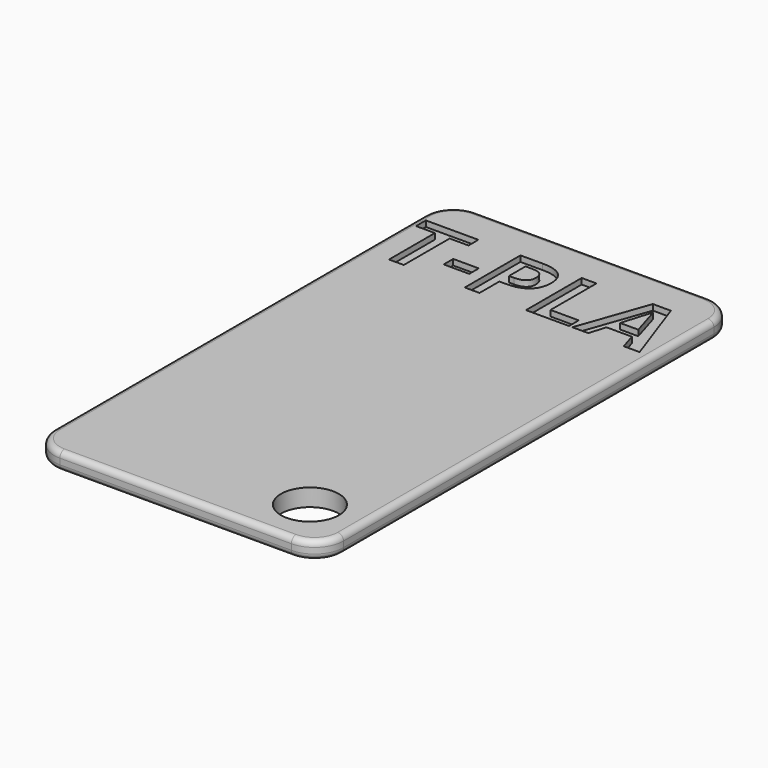
from build123d import *

# Parameters (mm, degrees)
F0_W         = 90
F0_H         = 50
F1_DEPTH     = 3
F2_R         = 1
F3_T1_DEPTH  = 3
F3_T4_ANGLE  = 90
F3_T6_ANGLE  = 90
F3_T8_ANGLE  = 90
F3_T10_ANGLE = 90
F3_T12_ANGLE = 90
F3_T14_ANGLE = 90
F3_T16_ANGLE = 90
F3_T18_ANGLE = 90
F5_ANGLE     = 90
F6_TEXT_SIZE = 16.8504196149
F7_DEPTH     = 1
F8_R         = 5
F9_DEPTH     = 3


# Not quite as in the source:
# - a fillet or chamfer that OpenCascade refuses, or shapes differently, is made with other operations: its cross-section is extruded or revolved along the edge and cut away or added
# - Text() gives the source's letters only with a copy of the font that has no kerning and outlines rounded to 1/6400 em; it was checked with that copy


with BuildPart() as f1:
    # F0 (on Top) → F1 (new body)
    with BuildSketch(Plane.XY):
        Rectangle(F0_W, F0_H)
    extrude(amount=F1_DEPTH)

    # F2
    f2_edges = [f1.edges().sort_by_distance(p)[0] for p in [
        (0, 25, 3),
        (-45, 0, 3),
        (0, -25, 3),
        (45, 0, 3),
        (0, 25, 0),
        (-45, 0, 0),
        (0, -25, 0),
        (45, 0, 0),
    ]]
    fillet(f2_edges, radius=F2_R)

    # F3: fillet of radius 5 on 4 edges, made by hand

    # F3_s2 → F3_t1 (cut)
    with BuildSketch(Plane.XY):
        with BuildLine():
            ThreePointArc((45, -20), (43.5355339059, -23.5355339059), (40, -25))
            Line((40, -25), (45, -25))
            Line((45, -25), (45, -20))
        make_face()
        with BuildLine():
            ThreePointArc((40, 25), (43.5355339059, 23.5355339059), (45, 20))
            Line((45, 20), (45, 25))
            Line((45, 25), (40, 25))
        make_face()
        with BuildLine():
            ThreePointArc((-40, 25), (-43.5355339059, 23.5355339059), (-45, 20))
            Line((-45, 20), (-45, 25))
            Line((-45, 25), (-40, 25))
        make_face()
        with BuildLine():
            ThreePointArc((-45, -20), (-43.5355339059, -23.5355339059), (-40, -25))
            Line((-40, -25), (-45, -25))
            Line((-45, -25), (-45, -20))
        make_face()
    extrude(amount=F3_T1_DEPTH, mode=Mode.SUBTRACT)

    # F3_s3 → F3_t4 (revolve, cut)
    with BuildSketch(Plane.YZ.offset(-40)):
        with BuildLine():
            ThreePointArc((-24, 0), (-24.7071067812, 0.2928932188), (-25, 1))
            Line((-25, 1), (-25, 0))
            Line((-25, 0), (-24, 0))
        make_face()
    revolve(axis=Axis((-40, -20, 0), (0, 0, -1)), revolution_arc=F3_T4_ANGLE, mode=Mode.SUBTRACT)

    # F3_s5 → F3_t6 (revolve, cut)
    with BuildSketch(Plane.XZ.offset(20)):
        with BuildLine():
            ThreePointArc((-44, 3), (-44.7071067812, 2.7071067812), (-45, 2))
            Line((-45, 2), (-45, 3))
            Line((-45, 3), (-44, 3))
        make_face()
    revolve(axis=Axis((-40, -20, 3), (0, 0, 1)), revolution_arc=F3_T6_ANGLE, mode=Mode.SUBTRACT)

    # F3_s7 → F3_t8 (revolve, cut)
    with BuildSketch(Plane.XZ.offset(-20)):
        with BuildLine():
            ThreePointArc((-44, 0), (-44.7071067812, 0.2928932188), (-45, 1))
            Line((-45, 1), (-45, 0))
            Line((-45, 0), (-44, 0))
        make_face()
    revolve(axis=Axis((-40, 20, 0), (0, 0, -1)), revolution_arc=F3_T8_ANGLE, mode=Mode.SUBTRACT)

    # F3_s9 → F3_t10 (revolve, cut)
    with BuildSketch(Plane.YZ.offset(-40)):
        with BuildLine():
            ThreePointArc((24, 3), (24.7071067812, 2.7071067812), (25, 2))
            Line((25, 2), (25, 3))
            Line((25, 3), (24, 3))
        make_face()
    revolve(axis=Axis((-40, 20, 3), (0, 0, 1)), revolution_arc=F3_T10_ANGLE, mode=Mode.SUBTRACT)

    # F3_s11 → F3_t12 (revolve, cut)
    with BuildSketch(Plane.YZ.offset(40)):
        with BuildLine():
            ThreePointArc((24, 0), (24.7071067812, 0.2928932188), (25, 1))
            Line((25, 1), (25, 0))
            Line((25, 0), (24, 0))
        make_face()
    revolve(axis=Axis((40, 20, 0), (0, 0, -1)), revolution_arc=F3_T12_ANGLE, mode=Mode.SUBTRACT)

    # F3_s13 → F3_t14 (revolve, cut)
    with BuildSketch(Plane.XZ.offset(-20)):
        with BuildLine():
            ThreePointArc((44, 3), (44.7071067812, 2.7071067812), (45, 2))
            Line((45, 2), (45, 3))
            Line((45, 3), (44, 3))
        make_face()
    revolve(axis=Axis((40, 20, 3), (0, 0, 1)), revolution_arc=F3_T14_ANGLE, mode=Mode.SUBTRACT)

    # F3_s15 → F3_t16 (revolve, cut)
    with BuildSketch(Plane.XZ.offset(20)):
        with BuildLine():
            ThreePointArc((44, 0), (44.7071067812, 0.2928932188), (45, 1))
            Line((45, 1), (45, 0))
            Line((45, 0), (44, 0))
        make_face()
    revolve(axis=Axis((40, -20, 0), (0, 0, -1)), revolution_arc=F3_T16_ANGLE, mode=Mode.SUBTRACT)

    # F3_s17 → F3_t18 (revolve, cut)
    with BuildSketch(Plane.YZ.offset(40)):
        with BuildLine():
            ThreePointArc((-24, 3), (-24.7071067812, 2.7071067812), (-25, 2))
            Line((-25, 2), (-25, 3))
            Line((-25, 3), (-24, 3))
        make_face()
    revolve(axis=Axis((40, -20, 3), (0, 0, 1)), revolution_arc=F3_T18_ANGLE, mode=Mode.SUBTRACT)


with BuildPart() as f1_1:
    # F5: moved
    add(f1.part.rotate(Axis((0, 0, 16.4477843791), (0, 0, 1)), F5_ANGLE))

    # F6 (on face) → F7 (cut)
    with BuildSketch(Plane.XY.offset(3)):
        with Locations((-24, 26.5792197825)):
            Text('T-PLA', F6_TEXT_SIZE, font='Open Sans', font_style=FontStyle.BOLD, text_align=(TextAlign.LEFT, TextAlign.BOTTOM))
    extrude(amount=-F7_DEPTH, mode=Mode.SUBTRACT)

    # F8 (on face) → F9 (cut)
    with BuildSketch(Plane.XY.offset(3)):
        with Locations((16, -36)):
            Circle(F8_R)
    extrude(amount=-F9_DEPTH, mode=Mode.SUBTRACT)


solid = f1_1.part
